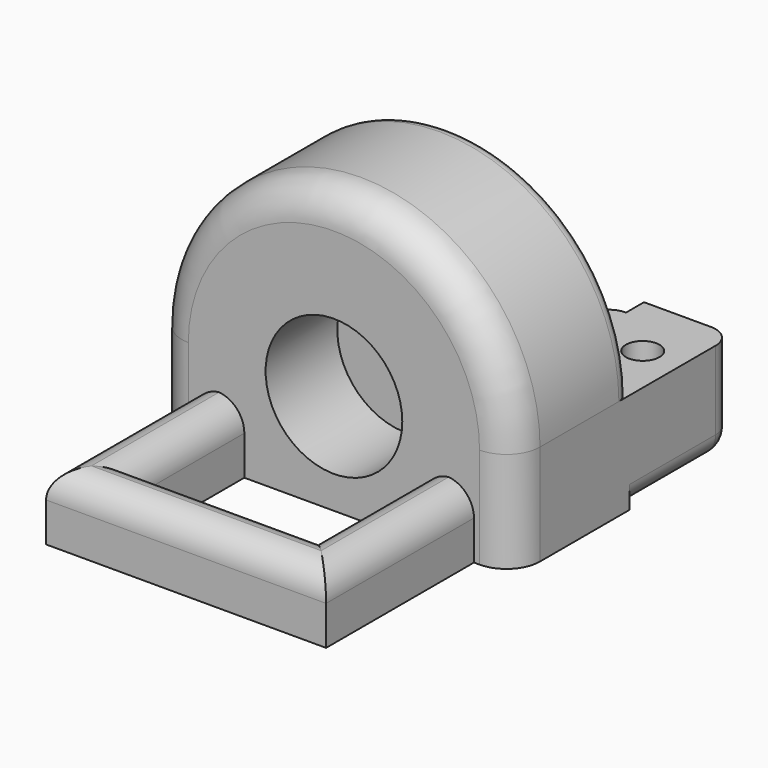
from build123d import *

# Parameters (mm, degrees)
F0_W          = 32
F0_H          = 11.6
F0_R          = 1.5
F1_DEPTH      = 9
F2_R          = 8
F1_FACE1_W    = 32
F1_FACE1_H    = 9
F3_DEPTH      = 5
F4_R          = 8
F5_DEPTH      = 2
F6_R          = 6
F7_DEPTH      = 25
F8_T1_DEPTH   = 28
F8_T3_DEPTH   = 12
F8_T5_DEPTH   = 14.6
F8_S9_W       = 2
F8_S9_H       = 2
F8_T10_DEPTH  = 2
F8_S15_W      = 2
F8_S15_H      = 2
F8_T16_DEPTH  = 2
F8_T20_ANGLE  = 275.6465366004
F10_DEPTH     = 13
F12_DEPTH     = 6
F13_T1_DEPTH  = 12
F13_T3_DEPTH  = 22.75
F13_T5_DEPTH  = 16
F13_T7_DEPTH  = 37.5
F13_T13_DEPTH = 18.25
F13_T17_DEPTH = 22.25
F13_T24_DEPTH = 18.25
F13_T28_DEPTH = 22.25
F14_R         = 3
F15_R         = 1.2
F16_R         = 6.1
F17_DEPTH     = 8
F18_T3_ANGLE  = 90
F18_T6_DEPTH  = 15
F18_T9_DEPTH  = 0.5
F19_R         = 2.1
F20_DEPTH     = 7


# Not quite as in the source:
# - a fillet or chamfer that OpenCascade refuses, or shapes differently, is made with other operations: its cross-section is extruded or revolved along the edge and cut away or added


with BuildPart() as f1:
    # F0 (on Top) → F1 (new body)
    with BuildSketch(Plane.XY):
        Rectangle(F0_W, F0_H)
        with Locations((-12.524, 0)):
            Circle(F0_R, mode=Mode.SUBTRACT)
        with Locations((12.524, 0)):
            Circle(F0_R, mode=Mode.SUBTRACT)
    extrude(amount=F1_DEPTH)

    # F2 (on face) + F1_face1 (on face) → F3 (cut)
    with BuildSketch(Plane.XZ.offset(5.8)):
        with Locations((0, 9)):
            Circle(F2_R)
    with BuildSketch(Plane(origin=(0, 5.8, 4.5), x_dir=(-1, 0, 0), z_dir=(0, 1, 0))):
        Rectangle(F1_FACE1_W, F1_FACE1_H)
    extrude(amount=-F3_DEPTH, dir=(0, -1, 0), mode=Mode.SUBTRACT)

    # F4 (on face) → F5 (cut)
    with BuildSketch(Plane(origin=(0, 5.8, 0), x_dir=(-1, 0, 0), z_dir=(0, 1, 0))):
        with Locations((0, 9)):
            Circle(F4_R)
    extrude(amount=-F5_DEPTH, mode=Mode.SUBTRACT)

    # F6 (on face) → F7 (cut)
    with BuildSketch(Plane(origin=(0, 3.8, 0), x_dir=(-1, 0, 0), z_dir=(0, 1, 0))):
        with Locations((0, 9)):
            Circle(F6_R)
    extrude(amount=-F7_DEPTH, mode=Mode.SUBTRACT)

    # F8: fillet of radius 2 on 6 edges, made by hand

    # F8_s2 → F8_t1 (cut)
    with BuildSketch(Plane.YZ.offset(-14)):
        with BuildLine():
            ThreePointArc((5.8, 2), (5.2142135624, 0.5857864376), (3.8, 0))
            Line((3.8, 0), (5.8, 0))
            Line((5.8, 0), (5.8, 2))
        make_face()
    extrude(amount=F8_T1_DEPTH, mode=Mode.SUBTRACT)

    # F8_s4 → F8_t3 (cut)
    with BuildSketch(Plane.XY.offset(2)):
        with BuildLine():
            ThreePointArc((-14, 5.8), (-15.4142135624, 5.2142135624), (-16, 3.8))
            Line((-16, 3.8), (-16, 5.8))
            Line((-16, 5.8), (-14, 5.8))
        make_face()
        with BuildLine():
            ThreePointArc((14, 5.8), (15.4142135624, 5.2142135624), (16, 3.8))
            Line((16, 3.8), (16, 5.8))
            Line((16, 5.8), (14, 5.8))
        make_face()
    extrude(amount=F8_T3_DEPTH, mode=Mode.SUBTRACT)

    # F8_s6 → F8_t5 (cut)
    with BuildSketch(Plane.XZ.offset(-3.8)):
        with BuildLine():
            ThreePointArc((-14, 0), (-15.4142135624, 0.5857864376), (-16, 2))
            Line((-16, 2), (-16, 0))
            Line((-16, 0), (-14, 0))
        make_face()
        with BuildLine():
            ThreePointArc((14, 0), (15.4142135624, 0.5857864376), (16, 2))
            Line((16, 2), (16, 0))
            Line((16, 0), (14, 0))
        make_face()
    extrude(amount=F8_T5_DEPTH, mode=Mode.SUBTRACT)


with BuildPart() as f8_tool8:
    # F8_s9 → F8_t10 (new body)
    with BuildSketch(Plane.XZ.offset(-3.8)):
        with Locations((15, 1)):
            Rectangle(F8_S9_W, F8_S9_H)
    extrude(amount=-F8_T10_DEPTH)

    # F8_s11 → F8_t12 (revolve, cut)
    with BuildSketch(Plane(origin=(14, 3.8, 2), x_dir=(-0.7071067812, 0, 0.7071067812), z_dir=(-0.7071067812, 0, -0.7071067812))):
        with BuildLine():
            ThreePointArc((0, -2), (2, 0), (0, 2))
            Line((0, 2), (0, -2))
        make_face()
    revolve(axis=Axis((14, 3.8, 2), (0, 1, 0)), mode=Mode.SUBTRACT)


with BuildPart() as f1_1:
    add(f1.part)

    # F8_t7: cut F8_tool8
    add(f8_tool8.part, mode=Mode.SUBTRACT)


with BuildPart() as f8_tool14:
    # F8_s15 → F8_t16 (new body)
    with BuildSketch(Plane.XZ.offset(-3.8)):
        with Locations((-15, 1)):
            Rectangle(F8_S15_W, F8_S15_H)
    extrude(amount=-F8_T16_DEPTH)

    # F8_s17 → F8_t18 (revolve, cut)
    with BuildSketch(Plane(origin=(-14, 3.8, 2), x_dir=(0.7071067812, 0, 0.7071067812), z_dir=(-0.7071067812, 0, 0.7071067812))):
        with BuildLine():
            ThreePointArc((0, -2), (2, 0), (0, 2))
            Line((0, 2), (0, -2))
        make_face()
    revolve(axis=Axis((-14, 3.8, 2), (0, 1, 0)), mode=Mode.SUBTRACT)


with BuildPart() as f1_2:
    add(f1_1.part)

    # F8_t13: cut F8_tool14
    add(f8_tool14.part, mode=Mode.SUBTRACT)

    # F8_s19 → F8_t20 (revolve, cut)
    with BuildSketch(Plane(origin=(-4.4781651596, 0, 4.057239564), x_dir=(0, 1, 0), z_dir=(-0.7410773266, 0, 0.6714196869))):
        with BuildLine():
            ThreePointArc((3.8, -14.6696959394), (3.2142135624, -13.255482377), (1.8, -12.6696959394))
            Line((1.8, -12.6696959394), (3.8, -12.6696959394))
            Line((3.8, -12.6696959394), (3.8, -14.6696959394))
        make_face()
    revolve(axis=Axis((0, 3.8, 9), (0, 1, 0)), revolution_arc=F8_T20_ANGLE, mode=Mode.SUBTRACT)

    # F9 (on face) → F10 (join)
    with BuildSketch(Plane.XZ.offset(5.8)):
        with BuildLine():
            Line((16, 0), (16, 9))
            ThreePointArc((16, 9), (0, 25), (-16, 9))
            Line((-16, 9), (-16, 0))
            Line((-16, 0), (-13.2287565553, 0))
            Line((-13.2287565553, 0), (0, 0))
            Line((0, 0), (13.2287565553, 0))
            Line((13.2287565553, 0), (16, 0))
        make_face()
    extrude(amount=F10_DEPTH)

    # F11 (on Top) → F12 (join)
    with BuildSketch(Plane.XY):
        Polygon((-8, -30.8), (-8, -18.8), (-12.5, -18.8), (-12.5, -35.3), (12.5, -35.3), (12.5, -18.8), (8, -18.8), (8, -30.8), align=None)
    extrude(amount=F12_DEPTH)

    # F13: fillet of radius 2.5 on 6 edges, made by hand

    # F13_s2 → F13_t1 (cut)
    with BuildSketch(Plane.XZ.offset(18.8)):
        with BuildLine():
            ThreePointArc((-10.5, 6), (-8.732233047, 5.267766953), (-8, 3.5))
            Line((-8, 3.5), (-8, 6))
            Line((-8, 6), (-10.5, 6))
        make_face()
        with BuildLine():
            ThreePointArc((10.5, 6), (8.732233047, 5.267766953), (8, 3.5))
            Line((8, 3.5), (8, 6))
            Line((8, 6), (10.5, 6))
        make_face()
    extrude(amount=F13_T1_DEPTH, mode=Mode.SUBTRACT)

    # F13_s4 → F13_t3 (cut)
    with BuildSketch(Plane.XZ.offset(18.8)):
        with BuildLine():
            ThreePointArc((-10, 6), (-11.767766953, 5.267766953), (-12.5, 3.5))
            Line((-12.5, 3.5), (-12.5, 6))
            Line((-12.5, 6), (-10, 6))
        make_face()
        with BuildLine():
            ThreePointArc((12.5, 3.5), (11.767766953, 5.267766953), (10, 6))
            Line((10, 6), (12.5, 6))
            Line((12.5, 6), (12.5, 3.5))
        make_face()
    extrude(amount=F13_T3_DEPTH, mode=Mode.SUBTRACT)

    # F13_s6 → F13_t5 (cut)
    with BuildSketch(Plane.YZ.offset(-8)):
        with BuildLine():
            ThreePointArc((-33.3, 6), (-31.532233047, 5.267766953), (-30.8, 3.5))
            Line((-30.8, 3.5), (-30.8, 6))
            Line((-30.8, 6), (-33.3, 6))
        make_face()
    extrude(amount=F13_T5_DEPTH, mode=Mode.SUBTRACT)

    # F13_s8 → F13_t7 (cut)
    with BuildSketch(Plane.YZ.offset(-18.75)):
        with BuildLine():
            ThreePointArc((-32.8, 6), (-34.567766953, 5.267766953), (-35.3, 3.5))
            Line((-35.3, 3.5), (-35.3, 6))
            Line((-35.3, 6), (-32.8, 6))
        make_face()
    extrude(amount=F13_T7_DEPTH, mode=Mode.SUBTRACT)


with BuildPart() as f13_tool11:
    # F13_s12 → F13_t13 (new body)
    with BuildSketch(Plane.XZ.offset(37.05)):
        with BuildLine():
            ThreePointArc((-10.5, 6), (-8.732233047, 5.267766953), (-8, 3.5))
            Line((-8, 3.5), (-8, 6))
            Line((-8, 6), (-10.5, 6))
        make_face()
    extrude(amount=-F13_T13_DEPTH)

    split(bisect_by=Plane.XZ.offset(30.8), keep=Keep.TOP)


with BuildPart() as f13_tool15:
    # F13_s16 → F13_t17 (new body)
    with BuildSketch(Plane.YZ.offset(8)):
        with BuildLine():
            ThreePointArc((-33.3, 6), (-31.532233047, 5.267766953), (-30.8, 3.5))
            Line((-30.8, 3.5), (-30.8, 6))
            Line((-30.8, 6), (-33.3, 6))
        make_face()
    extrude(amount=-F13_T17_DEPTH)

    split(bisect_by=Plane.YZ.offset(-8), keep=Keep.BOTTOM)


with BuildPart() as f13_tool11_1:
    add(f13_tool11.part)

    # F13_t19: intersect F13_tool15
    add(f13_tool15.part, mode=Mode.INTERSECT)


with BuildPart() as f1_3:
    add(f1_2.part)

    # F13_t9: cut F13_tool11
    add(f13_tool11_1.part, mode=Mode.SUBTRACT)


with BuildPart() as f13_tool22:
    # F13_s23 → F13_t24 (new body)
    with BuildSketch(Plane.XZ.offset(18.8)):
        with BuildLine():
            ThreePointArc((10.5, 6), (8.732233047, 5.267766953), (8, 3.5))
            Line((8, 3.5), (8, 6))
            Line((8, 6), (10.5, 6))
        make_face()
    extrude(amount=F13_T24_DEPTH)

    split(bisect_by=Plane.XZ.offset(30.8), keep=Keep.TOP)


with BuildPart() as f13_tool26:
    # F13_s27 → F13_t28 (new body)
    with BuildSketch(Plane.YZ.offset(14.25)):
        with BuildLine():
            ThreePointArc((-33.3, 6), (-31.532233047, 5.267766953), (-30.8, 3.5))
            Line((-30.8, 3.5), (-30.8, 6))
            Line((-30.8, 6), (-33.3, 6))
        make_face()
    extrude(amount=-F13_T28_DEPTH)

    split(bisect_by=Plane.YZ.offset(8), keep=Keep.TOP)


with BuildPart() as f13_tool22_1:
    add(f13_tool22.part)

    # F13_t30: intersect F13_tool26
    add(f13_tool26.part, mode=Mode.INTERSECT)


with BuildPart() as f1_4:
    add(f1_3.part)

    # F13_t20: cut F13_tool22
    add(f13_tool22_1.part, mode=Mode.SUBTRACT)

    # F14
    f14_edges = [f1_4.edges().sort_by_distance(p)[0] for p in [
        (0, -18.8, 25),
        (16, -18.8, 4.5),
    ]]
    fillet(f14_edges, radius=F14_R)

    # F15
    f15_edges = [f1_4.edges().sort_by_distance(p)[0] for p in [
        (0, -5.8, 25),
    ]]
    fillet(f15_edges, radius=F15_R)

    # F16 (on face) → F17 (cut)
    with BuildSketch(Plane.XZ.offset(18.8)):
        with Locations((0, 9)):
            Circle(F16_R)
    extrude(amount=-F17_DEPTH, mode=Mode.SUBTRACT)

    # F18: fillet of radius 2 on 3 edges, made by hand


with BuildPart() as f18_tool1:
    # F18_s2 → F18_t3 (revolve)
    with BuildSketch(Plane.XZ.offset(15.8)):
        with BuildLine():
            ThreePointArc((-16, 2), (-15.4142135624, 0.5857864376), (-14, 0))
            Line((-14, 0), (-16, 0))
            Line((-16, 0), (-16, 2))
        make_face()
    revolve(axis=Axis((-13, -15.8, 0), (0, 0, 1)), revolution_arc=F18_T3_ANGLE)


with BuildPart() as f18_tool4:
    # F18_s5 → F18_t6 (new body)
    with BuildSketch(Plane.XZ.offset(0.8)):
        with BuildLine():
            ThreePointArc((-16, 2), (-15.4142135624, 0.5857864376), (-14, 0))
            Line((-14, 0), (-16, 0))
            Line((-16, 0), (-16, 2))
        make_face()
    extrude(amount=F18_T6_DEPTH)


with BuildPart() as f18_tool7:
    # F18_s8 → F18_t9 (new body)
    with BuildSketch(Plane.YZ.offset(-12.5)):
        with BuildLine():
            ThreePointArc((-18.8, 2), (-18.2142135624, 0.5857864376), (-16.8, 0))
            Line((-16.8, 0), (-18.8, 0))
            Line((-18.8, 0), (-18.8, 2))
        make_face()
    extrude(amount=-F18_T9_DEPTH)


with BuildPart() as f1_5:
    add(f1_4.part)

    # F18_t10: cut F18_tool1, F18_tool4, F18_tool7
    add([f18_tool1.part, f18_tool4.part, f18_tool7.part], mode=Mode.SUBTRACT)

    # F19 (on face) → F20 (cut)
    with BuildSketch(Plane(origin=(0, -5.8, 0), x_dir=(-1, 0, 0), z_dir=(0, 1, 0))):
        with Locations((0, 9)):
            Circle(F19_R)
    extrude(amount=-F20_DEPTH, mode=Mode.SUBTRACT)


solid = f1_5.part
